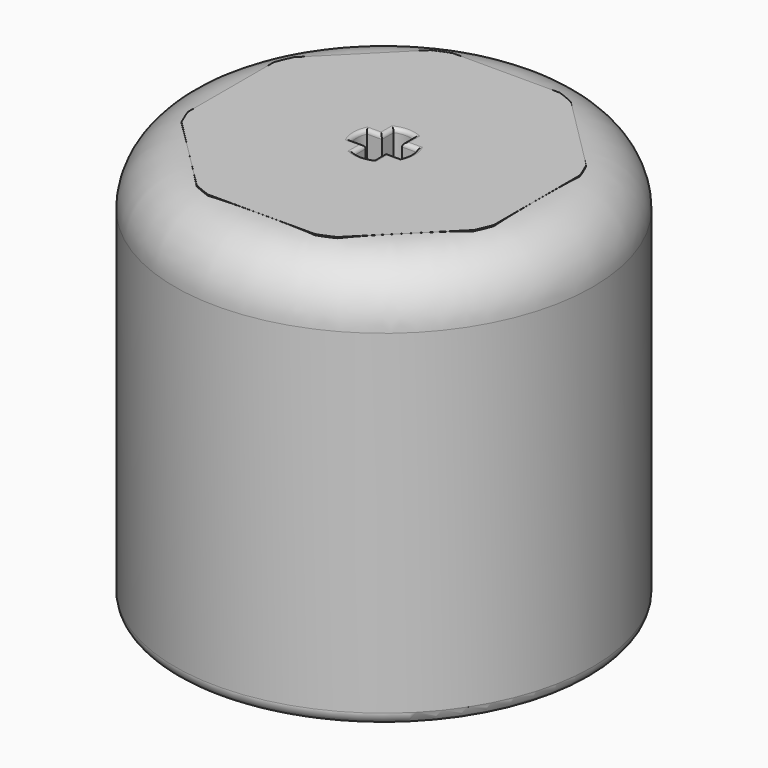
from build123d import *

# Parameters (mm, degrees)
F1_START = 25.4
F1_DEPTH = 2.54
F2_START = 25.4
F0_R     = 6.35
F2_DEPTH = 15.24
F3_START = 25.4
F3_DEPTH = 15.24
F0_R_2   = 20.955
F4_DEPTH = 40.64
F5_R     = 0.381
F7_R     = 1.27


# Not quite as in the source:
# - a fillet or chamfer that OpenCascade refuses, or shapes differently, is made with other operations: its cross-section is extruded or revolved along the edge and cut away or added
# - a feature names something its author has since deleted; it is built from what else it names


with BuildPart() as f1:
    # F0 (on Top) → F1 (new body)
    with BuildSketch(Plane.XY.offset(F1_START)):
        with BuildLine():
            Line((-40.3893615403, 31.7689274535), (-38.8988945509, 31.7689274535))
            Line((-38.8988945509, 31.7689274535), (-38.8988945509, 30.2784604641))
            ThreePointArc((-38.8988945509, 30.2784604641), (-37.8863945509, 30.0814274535), (-36.8738945509, 30.2784604641))
            Line((-36.8738945509, 30.2784604641), (-36.8738945509, 31.7689274535))
            Line((-36.8738945509, 31.7689274535), (-35.3834275615, 31.7689274535))
            ThreePointArc((-35.3834275615, 31.7689274535), (-35.1863945509, 32.7814274535), (-35.3834275615, 33.7939274535))
            Line((-35.3834275615, 33.7939274535), (-36.8738945509, 33.7939274535))
            Line((-36.8738945509, 33.7939274535), (-36.8738945509, 35.2843944429))
            ThreePointArc((-36.8738945509, 35.2843944429), (-37.8863945509, 35.4814274535), (-38.8988945509, 35.2843944429))
            Line((-38.8988945509, 35.2843944429), (-38.8988945509, 33.7939274535))
            Line((-38.8988945509, 33.7939274535), (-40.3893615403, 33.7939274535))
            ThreePointArc((-40.3893615403, 33.7939274535), (-40.5863945509, 32.7814274535), (-40.3893615403, 31.7689274535))
        make_face()
    extrude(amount=F1_DEPTH)

    # F0 (on Top) → F2 (join)
    with BuildSketch(Plane.XY.offset(F2_START)):
        with Locations((-37.8863945509, 32.7814274535)):
            Circle(F0_R)
        with BuildLine():
            Line((-38.8988945509, 30.2784604641), (-38.8988945509, 31.7689274535))
            Line((-38.8988945509, 31.7689274535), (-40.3893615403, 31.7689274535))
            ThreePointArc((-40.3893615403, 31.7689274535), (-40.5863945509, 32.7814274535), (-40.3893615403, 33.7939274535))
            Line((-40.3893615403, 33.7939274535), (-38.8988945509, 33.7939274535))
            Line((-38.8988945509, 33.7939274535), (-38.8988945509, 35.2843944429))
            ThreePointArc((-38.8988945509, 35.2843944429), (-37.8863945509, 35.4814274535), (-36.8738945509, 35.2843944429))
            Line((-36.8738945509, 35.2843944429), (-36.8738945509, 33.7939274535))
            Line((-36.8738945509, 33.7939274535), (-35.3834275615, 33.7939274535))
            ThreePointArc((-35.3834275615, 33.7939274535), (-35.1863945509, 32.7814274535), (-35.3834275615, 31.7689274535))
            Line((-35.3834275615, 31.7689274535), (-36.8738945509, 31.7689274535))
            Line((-36.8738945509, 31.7689274535), (-36.8738945509, 30.2784604641))
            ThreePointArc((-36.8738945509, 30.2784604641), (-37.8863945509, 30.0814274535), (-38.8988945509, 30.2784604641))
        make_face(mode=Mode.SUBTRACT)
    extrude(amount=F2_DEPTH)

    # F0 (on Top) → F3 (join)
    with BuildSketch(Plane.XY.offset(F3_START)):
        with BuildLine():
            Line((-22.5447945509, 27.4062209049), (-22.5447945509, 38.1566340021))
            ThreePointArc((-22.5447945509, 38.1566340021), (-22.8678088704, 39.00232933), (-23.2374001559, 39.8287318469))
            Line((-23.2374001559, 39.8287318469), (-30.8390901575, 47.4304218485))
            ThreePointArc((-30.8390901575, 47.4304218485), (-31.6654926744, 47.800013134), (-32.5111880023, 48.1230274535))
            Line((-32.5111880023, 48.1230274535), (-43.2616010995, 48.1230274535))
            ThreePointArc((-43.2616010995, 48.1230274535), (-44.1072964275, 47.800013134), (-44.9336989444, 47.4304218485))
            Line((-44.9336989444, 47.4304218485), (-52.535388946, 39.8287318469))
            ThreePointArc((-52.535388946, 39.8287318469), (-52.9049802314, 39.00232933), (-53.2279945509, 38.1566340021))
            Line((-53.2279945509, 38.1566340021), (-53.2279945509, 27.4062209049))
            ThreePointArc((-53.2279945509, 27.4062209049), (-52.9049802314, 26.5605255769), (-52.535388946, 25.73412306))
            Line((-52.535388946, 25.73412306), (-44.9336989444, 18.1324330584))
            ThreePointArc((-44.9336989444, 18.1324330584), (-44.1072964275, 17.762841773), (-43.2616010995, 17.4398274535))
            Line((-43.2616010995, 17.4398274535), (-32.5111880023, 17.4398274535))
            ThreePointArc((-32.5111880023, 17.4398274535), (-31.6654926744, 17.762841773), (-30.8390901575, 18.1324330584))
            Line((-30.8390901575, 18.1324330584), (-23.2374001559, 25.73412306))
            ThreePointArc((-23.2374001559, 25.73412306), (-22.8678088704, 26.5605255769), (-22.5447945509, 27.4062209049))
        make_face()
        with Locations((-37.8863945509, 32.7814274535)):
            Circle(F0_R, mode=Mode.SUBTRACT)
    extrude(amount=F3_DEPTH)

    # F5
    f5_edges = [f1.edges().sort_by_distance(p)[0] for p in [
        (-36.128661, 33.793927, 40.64),
        (-35.186395, 32.781427, 40.64),
        (-36.873895, 31.023694, 40.64),
        (-36.873895, 34.539161, 40.64),
        (-37.886395, 35.481427, 40.64),
        (-36.128661, 31.768927, 40.64),
        (-39.644128, 33.793927, 40.64),
        (-38.898895, 34.539161, 40.64),
        (-39.644128, 31.768927, 40.64),
        (-40.586395, 32.781427, 40.64),
        (-38.898895, 31.023694, 40.64),
        (-37.886395, 30.081427, 40.64),
    ]]
    fillet(f5_edges, radius=F5_R)


with BuildPart() as f4:
    # F0 (on Top) → F4 (new body)
    with BuildSketch(Plane.XY):
        with Locations((-37.8863945509, 32.7814274535)):
            Circle(F0_R_2)
        with BuildLine():
            ThreePointArc((-23.2374001559, 39.8287318469), (-22.8678088704, 39.00232933), (-22.5447945509, 38.1566340021))
            Line((-22.5447945509, 38.1566340021), (-22.5447945509, 27.4062209049))
            ThreePointArc((-22.5447945509, 27.4062209049), (-22.8678088704, 26.5605255769), (-23.2374001559, 25.73412306))
            Line((-23.2374001559, 25.73412306), (-30.8390901575, 18.1324330584))
            ThreePointArc((-30.8390901575, 18.1324330584), (-31.6654926744, 17.762841773), (-32.5111880023, 17.4398274535))
            Line((-32.5111880023, 17.4398274535), (-43.2616010995, 17.4398274535))
            ThreePointArc((-43.2616010995, 17.4398274535), (-44.1072964275, 17.762841773), (-44.9336989444, 18.1324330584))
            Line((-44.9336989444, 18.1324330584), (-52.535388946, 25.73412306))
            ThreePointArc((-52.535388946, 25.73412306), (-52.9049802314, 26.5605255769), (-53.2279945509, 27.4062209049))
            Line((-53.2279945509, 27.4062209049), (-53.2279945509, 38.1566340021))
            ThreePointArc((-53.2279945509, 38.1566340021), (-52.9049802314, 39.00232933), (-52.535388946, 39.8287318469))
            Line((-52.535388946, 39.8287318469), (-44.9336989444, 47.4304218485))
            ThreePointArc((-44.9336989444, 47.4304218485), (-44.1072964275, 47.800013134), (-43.2616010995, 48.1230274535))
            Line((-43.2616010995, 48.1230274535), (-32.5111880023, 48.1230274535))
            ThreePointArc((-32.5111880023, 48.1230274535), (-31.6654926744, 47.800013134), (-30.8390901575, 47.4304218485))
            Line((-30.8390901575, 47.4304218485), (-23.2374001559, 39.8287318469))
        make_face(mode=Mode.SUBTRACT)
    extrude(amount=F4_DEPTH)

    # F6: fillet of radius 5.842 on 1 edges, made by hand

    # F6_s1 → F6_t2 (revolve, cut)
    with BuildSketch(Plane.XZ.offset(-32.7814274535)):
        with BuildLine():
            ThreePointArc((-16.9313945509, 34.798), (-18.6424767352, 38.9289178157), (-22.7733945509, 40.64))
            Line((-22.7733945509, 40.64), (-16.9313945509, 40.64))
            Line((-16.9313945509, 40.64), (-16.9313945509, 34.798))
        make_face()
    revolve(axis=Axis((-37.8863945509, 32.7814274535, 40.64), (0, 0, 1)), mode=Mode.SUBTRACT)

    # F7
    f7_edges = [f4.edges().sort_by_distance(p)[0] for p in [
        (-58.841395, 32.781427, 0),
        (-37.886395, 17.439827, 0),
        (-48.734544, 21.933278, 0),
        (-44.107296, 17.762842, 0),
        (-31.665493, 17.762842, 0),
        (-27.038245, 21.933278, 0),
        (-22.867809, 26.560526, 0),
        (-22.544795, 32.781427, 0),
        (-22.867809, 39.002329, 0),
        (-27.038245, 43.629577, 0),
        (-52.90498, 26.560526, 0),
        (-53.227995, 32.781427, 0),
        (-52.90498, 39.002329, 0),
        (-48.734544, 43.629577, 0),
        (-44.107296, 47.800013, 0),
        (-37.886395, 48.123027, 0),
        (-31.665493, 47.800013, 0),
    ]]
    fillet(f7_edges, radius=F7_R)


solid = Compound([f1.part, f4.part])
